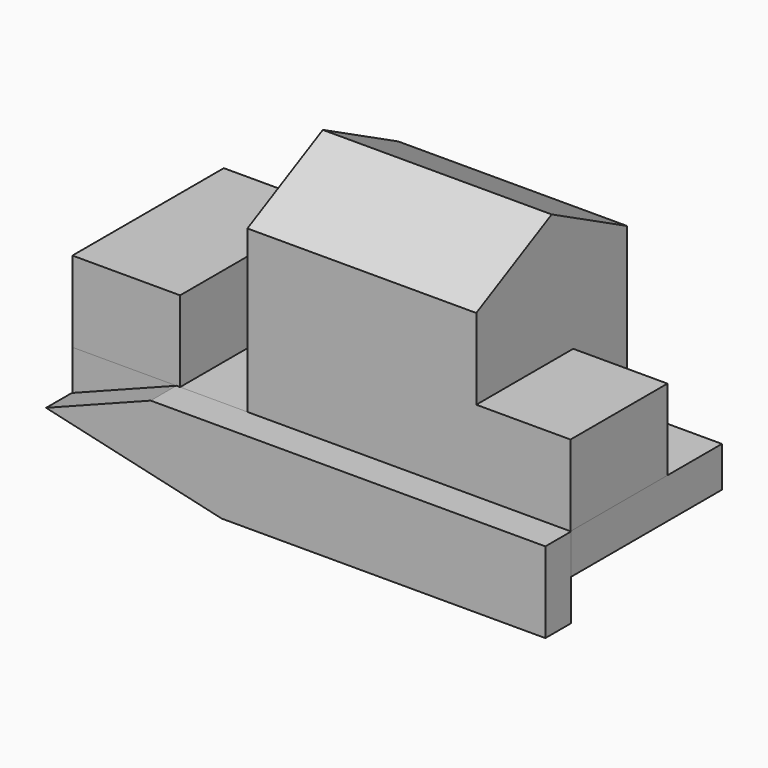
from build123d import *

# Parameters (mm, degrees)
F0_W      = 400
F0_H      = 702.9774785042
F1_DEPTH  = 300
F2_DEPTH  = 300
F4_DEPTH  = 300
F5_W      = 850
F5_H      = 350
F6_DEPTH  = 180
F8_DEPTH  = 1000
F9_DEPTH  = 180
F10_DEPTH = 180
F11_DEPTH = 1000
F13_DEPTH = 10000
F14_W     = 1854.3438315392
F14_H     = 119.6197420359
F15_DEPTH = 300
F17_DEPTH = 200
F18_DEPTH = 200
F19_W     = 400
F19_H     = 702.9774785042
F20_DEPTH = 150
F21_W     = 702.9774785042
F21_H     = 150
F22_DEPTH = 1450


# Not quite as in the source:
# - a feature of the source that left no trace in its solid (it failed there, or was rolled back) is left out
# - a feature names something its author has since deleted; it is built from what else it names


with BuildPart() as f1:
    # F0 (on Top) → F1 (new body)
    with BuildSketch(Plane.XY):
        with Locations((-450, 351.4887392521)):
            Rectangle(F0_W, F0_H)
    extrude(amount=F1_DEPTH)

    # F16 (on face) → F18 (cut)
    with BuildSketch(Plane.XZ.offset(119.6197420359)):
        Polygon((0, -300), (-652.1208882332, -150), (-652.1208882332, -300), align=None)
        Polygon((-652.1208882332, 0), (-652.1208882332, -150), (-263.4871304035, 0), align=None)
    extrude(amount=-F18_DEPTH, mode=Mode.SUBTRACT)


with BuildPart() as f2:
    # F0 (on Top) → F2 (new body)
    with BuildSketch(Plane.XY):
        Polygon((0, 700), (0, 0), (1200, 0), (1200, 150.83758533), (1200, 450), (850, 450), (850, 700), align=None)
    extrude(amount=F2_DEPTH)

    # F3 (on face) → F4 (join)
    with BuildSketch(Plane.XY.offset(300)):
        Polygon((0, 700), (0, 0), (850, 0), (850, 450), (850, 700), align=None)
    extrude(amount=F4_DEPTH)

    # F5 (on face) → F6 (join)
    with BuildSketch(Plane.XY.offset(600)):
        with Locations((425, 175)):
            Rectangle(F5_W, F5_H)
    extrude(amount=F6_DEPTH)

    # F7 (on face) → F8 (cut)
    with BuildSketch(Plane(origin=(0, 0, 0), x_dir=(0, -1, 0), z_dir=(-1, 0, 0))):
        Polygon((0, 780), (-350, 780), (0, 600), align=None)
    extrude(amount=-F8_DEPTH, mode=Mode.SUBTRACT)

    # F5 (on face) → F9 (join)
    with BuildSketch(Plane.XY.offset(600)):
        with Locations((425, 525)):
            Rectangle(F5_W, F5_H)
    extrude(amount=F9_DEPTH)

    # F5 (on face) → F10 (join)
    with BuildSketch(Plane.XY.offset(600)):
        with Locations((425, 525)):
            Rectangle(F5_W, F5_H)
        with Locations((425, 175)):
            Rectangle(F5_W, F5_H)
    extrude(amount=F10_DEPTH)

    # F7 (on face) → F11 (cut)
    with BuildSketch(Plane(origin=(0, 0, 0), x_dir=(0, -1, 0), z_dir=(-1, 0, 0))):
        Polygon((0, 780), (-350, 780), (0, 600), align=None)
    extrude(amount=-F11_DEPTH, mode=Mode.SUBTRACT)

    # F12 (on face) → F13 (cut)
    with BuildSketch(Plane(origin=(0, 0, 0), x_dir=(0, -1, 0), z_dir=(-1, 0, 0))):
        Polygon((-700, 600), (-350, 780), (-700, 780), align=None)
    extrude(amount=-F13_DEPTH, mode=Mode.SUBTRACT)


with BuildPart() as f15:
    # F14 (on Top) → F15 (new body)
    with BuildSketch(Plane.XY):
        with Locations((275.0510275364, -59.8098710179)):
            Rectangle(F14_W, F14_H)
    extrude(amount=-F15_DEPTH)

    # F16 (on face) → F17 (cut)
    with BuildSketch(Plane.XZ.offset(119.6197420359)):
        Polygon((0, -300), (-652.1208882332, -150), (-652.1208882332, -300), align=None)
        Polygon((-652.1208882332, 0), (-652.1208882332, -150), (-263.4871304035, 0), align=None)
    extrude(amount=-F17_DEPTH, mode=Mode.SUBTRACT)


with BuildPart() as f20:
    # F19 (on face) → F20 (new body)
    with BuildSketch(Plane(origin=(0, 0, 0), x_dir=(1, 0, 0), z_dir=(0, 0, -1))):
        with Locations((-450, -351.4887392521)):
            Rectangle(F19_W, F19_H)
    extrude(amount=F20_DEPTH)


with BuildPart() as f22:
    # F21 (on face) → F22 (new body)
    with BuildSketch(Plane.YZ.offset(-250)):
        with Locations((351.4887392521, -75)):
            Rectangle(F21_W, F21_H)
    extrude(amount=F22_DEPTH)


solid = Compound([f1.part, f2.part, f15.part, f20.part, f22.part])
